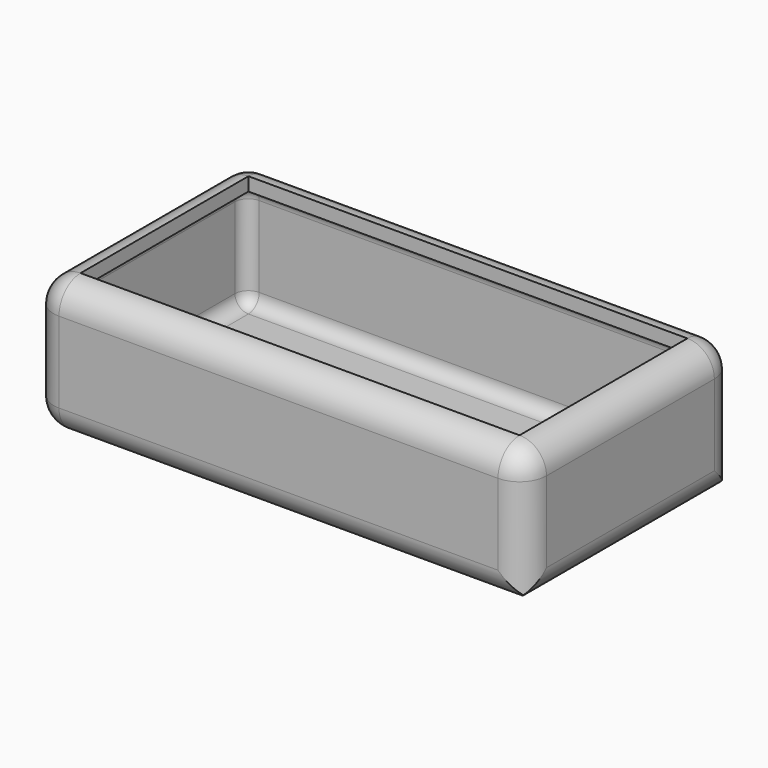
from build123d import *

# Parameters (mm, degrees)
F0_W         = 91.4515480399
F0_H         = 48.9329919219
F1_DEPTH     = 12.5
F2_R         = 5
F3_R         = 5
F4_T1_DEPTH  = 27.5
F4_T3_DEPTH  = 38.9329919219
F4_T5_DEPTH  = 81.4515480399
F4_S9_W      = 5.1
F4_S9_H      = 5.1
F4_T10_DEPTH = 5.1
F4_S15_W     = 5.1
F4_S15_H     = 5.1
F4_T16_DEPTH = 5.1
F4_T20_ANGLE = 90
F4_T22_ANGLE = 90
F5_T         = -2.5


# Not quite as in the source:
# - a fillet or chamfer that OpenCascade refuses, or shapes differently, is made with other operations: its cross-section is extruded or revolved along the edge and cut away or added
# - a shell that OpenCascade refuses in one call is made with other operations: the cavity is built on its own and cut out


with BuildPart() as f1:
    # F0 (on Top) → F1 (new body, symmetric)
    with BuildSketch(Plane.XY):
        with Locations((0.825881958, -0.5985237658)):
            Rectangle(F0_W, F0_H)
    extrude(amount=F1_DEPTH, both=True)

    # F2
    f2_edges = [f1.edges().sort_by_distance(p)[0] for p in [
        (-44.899892, 23.867972, 0),
    ]]
    fillet(f2_edges, radius=F2_R)

    # F3
    f3_edges = [f1.edges().sort_by_distance(p)[0] for p in [
        (-44.899892, -25.06502, 0),
        (3.325882, 23.867972, -12.5),
        (-43.435426, 22.403506, -12.5),
        (46.551656, -0.598524, -12.5),
        (-44.899892, -3.098524, -12.5),
        (0.825882, -25.06502, -12.5),
    ]]
    fillet(f3_edges, radius=F3_R)

    # F4: fillet of radius 5 on 9 edges, made by hand

    # F4_s2 → F4_t1 (cut)
    with BuildSketch(Plane.XY.offset(-20)):
        with BuildLine():
            ThreePointArc((41.551655978, 23.8679721951), (45.0871898839, 22.4035061011), (46.551655978, 18.8679721951))
            Line((46.551655978, 18.8679721951), (46.551655978, 23.8679721951))
            Line((46.551655978, 23.8679721951), (41.551655978, 23.8679721951))
        make_face()
        with BuildLine():
            ThreePointArc((46.551655978, -20.0650197268), (45.0871898839, -23.6005536327), (41.551655978, -25.0650197268))
            Line((41.551655978, -25.0650197268), (46.551655978, -25.0650197268))
            Line((46.551655978, -25.0650197268), (46.551655978, -20.0650197268))
        make_face()
    extrude(amount=F4_T1_DEPTH, mode=Mode.SUBTRACT)

    # F4_s4 → F4_t3 (cut)
    with BuildSketch(Plane.XZ.offset(-18.8679721951)):
        with BuildLine():
            ThreePointArc((41.551655978, 12.5), (45.0871898839, 11.0355339059), (46.551655978, 7.5))
            Line((46.551655978, 7.5), (46.551655978, 12.5))
            Line((46.551655978, 12.5), (41.551655978, 12.5))
        make_face()
        with BuildLine():
            ThreePointArc((-39.8998920619, 12.5), (-43.4354259679, 11.0355339059), (-44.8998920619, 7.5))
            Line((-44.8998920619, 7.5), (-44.8998920619, 12.5))
            Line((-44.8998920619, 12.5), (-39.8998920619, 12.5))
        make_face()
    extrude(amount=F4_T3_DEPTH, mode=Mode.SUBTRACT)

    # F4_s6 → F4_t5 (cut)
    with BuildSketch(Plane.YZ.offset(-39.8998920619)):
        with BuildLine():
            ThreePointArc((23.8679721951, 7.5), (22.4035061011, 11.0355339059), (18.8679721951, 12.5))
            Line((18.8679721951, 12.5), (23.8679721951, 12.5))
            Line((23.8679721951, 12.5), (23.8679721951, 7.5))
        make_face()
        with BuildLine():
            ThreePointArc((-20.0650197268, 12.5), (-23.6005536327, 11.0355339059), (-25.0650197268, 7.5))
            Line((-25.0650197268, 7.5), (-25.0650197268, 12.5))
            Line((-25.0650197268, 12.5), (-20.0650197268, 12.5))
        make_face()
    extrude(amount=F4_T5_DEPTH, mode=Mode.SUBTRACT)


with BuildPart() as f4_tool8:
    # F4_s9 → F4_t10 (new body)
    with BuildSketch(Plane.XZ.offset(-18.8679721951)):
        with Locations((44.101655978, 10.05)):
            Rectangle(F4_S9_W, F4_S9_H)
    extrude(amount=-F4_T10_DEPTH)

    # F4_s11 → F4_t12 (revolve, cut)
    with BuildSketch(Plane(origin=(41.551655978, 18.8679721951, 7.5), x_dir=(-0.7071067812, 0, -0.7071067812), z_dir=(0.7071067812, 0, -0.7071067812))):
        with BuildLine():
            ThreePointArc((0, -5), (5, 0), (0, 5))
            Line((0, 5), (0, -5))
        make_face()
    revolve(axis=Axis((41.551655978, 18.8679721951, 7.5), (0, 1, 0)), mode=Mode.SUBTRACT)


with BuildPart() as f1_1:
    add(f1.part)

    # F4_t7: cut F4_tool8
    add(f4_tool8.part, mode=Mode.SUBTRACT)


with BuildPart() as f4_tool14:
    # F4_s15 → F4_t16 (new body)
    with BuildSketch(Plane.XZ.offset(20.0650197268)):
        with Locations((44.101655978, 10.05)):
            Rectangle(F4_S15_W, F4_S15_H)
    extrude(amount=F4_T16_DEPTH)

    # F4_s17 → F4_t18 (revolve, cut)
    with BuildSketch(Plane(origin=(41.551655978, -20.0650197268, 7.5), x_dir=(-0.7071067812, 0, -0.7071067812), z_dir=(-0.7071067812, 0, 0.7071067812))):
        with BuildLine():
            ThreePointArc((0, -5), (5, 0), (0, 5))
            Line((0, 5), (0, -5))
        make_face()
    revolve(axis=Axis((41.551655978, -20.0650197268, 7.5), (0, -1, 0)), mode=Mode.SUBTRACT)


with BuildPart() as f1_2:
    add(f1_1.part)

    # F4_t13: cut F4_tool14
    add(f4_tool14.part, mode=Mode.SUBTRACT)

    # F4_s19 → F4_t20 (revolve, cut)
    with BuildSketch(Plane.YZ.offset(-39.8998920619)):
        with BuildLine():
            ThreePointArc((23.8679721951, 7.5), (22.4035061011, 11.0355339059), (18.8679721951, 12.5))
            Line((18.8679721951, 12.5), (23.8679721951, 12.5))
            Line((23.8679721951, 12.5), (23.8679721951, 7.5))
        make_face()
    revolve(axis=Axis((-39.8998920619, 18.8679721951, 12.5), (0, 0, 1)), revolution_arc=F4_T20_ANGLE, mode=Mode.SUBTRACT)

    # F4_s21 → F4_t22 (revolve, cut)
    with BuildSketch(Plane.XZ.offset(20.0650197268)):
        with BuildLine():
            ThreePointArc((-39.8998920619, 12.5), (-43.4354259679, 11.0355339059), (-44.8998920619, 7.5))
            Line((-44.8998920619, 7.5), (-44.8998920619, 12.5))
            Line((-44.8998920619, 12.5), (-39.8998920619, 12.5))
        make_face()
    revolve(axis=Axis((-39.8998920619, -20.0650197268, 12.5), (0, 0, 1)), revolution_arc=F4_T22_ANGLE, mode=Mode.SUBTRACT)

    # F5: a shell. OpenCascade refuses it in one call, so the cavity is built on its own and cut out:
    # the body offset inwards by the wall thickness, plus a prism from it out through each open face.
    f5_core = offset(f1_2.part, amount=F5_T, mode=Mode.PRIVATE)
    f5_exits = [f5_core.faces().sort_by_distance(p)[0] for p in [
        (0.825882, -0.598524, 10),
    ]]
    add(f5_core, mode=Mode.SUBTRACT)
    extrude(f5_exits, amount=-F5_T, mode=Mode.SUBTRACT)


solid = f1_2.part
